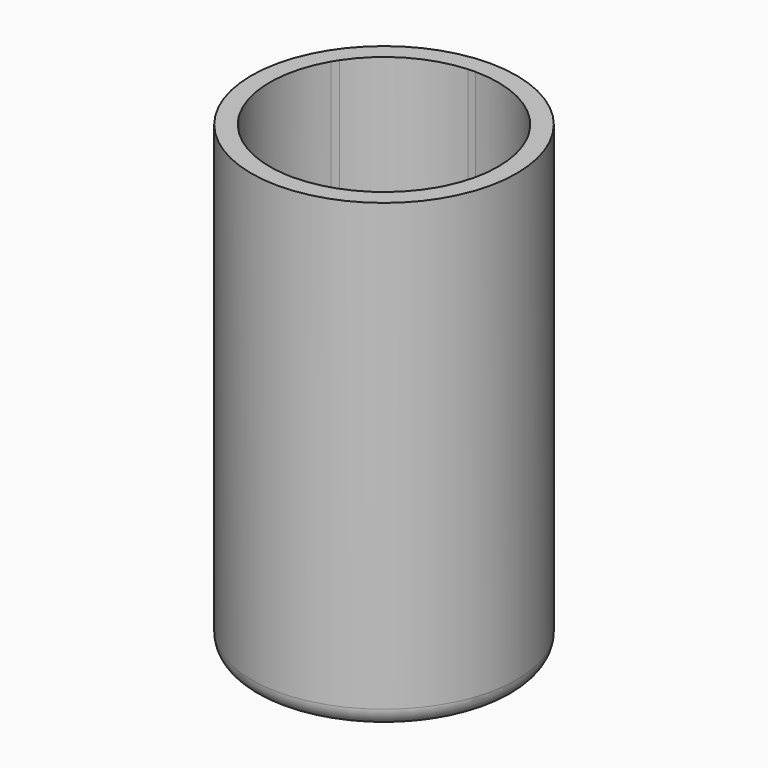
from build123d import *

# Parameters (mm, degrees)
F0_R     = 36
F1_DEPTH = 126
F2_DEPTH = 4
F3_R     = 5
F4_DEPTH = 10
F5_DEPTH = 5
F6_DEPTH = 5


# Not quite as in the source:
# - a feature names something its author has since deleted; it is built from what else it names


with BuildPart() as f1:
    # F0 (on Top) → F1 (new body)
    with BuildSketch(Plane.XY):
        Circle(F0_R)
        with BuildLine():
            ThreePointArc((27.7903944838, 13.7365925335), (30.1869361562, 7.0532889846), (31, 0))
            ThreePointArc((31, 0), (30.1869361562, -7.0532889846), (27.7903944838, -13.7365925335))
            ThreePointArc((27.7903944838, -13.7365925335), (27.33281573, -14.625907981), (26.8467875173, -15.5))
            ThreePointArc((26.8467875173, -15.5), (15.5, -26.8467875173), (0, -31))
            ThreePointArc((0, -31), (-1, -30.9838667697), (-1.9989591464, -30.935483871))
            ThreePointArc((-1.9989591464, -30.935483871), (-15.5, -26.8467875173), (-25.7914353374, -17.1988913374))
            ThreePointArc((-25.7914353374, -17.1988913374), (-26.33281573, -16.3579587886), (-26.8467875173, -15.5))
            ThreePointArc((-26.8467875173, -15.5), (-31, 0), (-26.8467875173, 15.5))
            ThreePointArc((-26.8467875173, 15.5), (-26.33281573, 16.3579587886), (-25.7914353374, 17.1988913374))
            ThreePointArc((-25.7914353374, 17.1988913374), (-15.5, 26.8467875173), (-1.9989591464, 30.935483871))
            ThreePointArc((-1.9989591464, 30.935483871), (-1, 30.9838667697), (0, 31))
            ThreePointArc((0, 31), (15.5, 26.8467875173), (26.8467875173, 15.5))
            ThreePointArc((26.8467875173, 15.5), (27.33281573, 14.625907981), (27.7903944838, 13.7365925335))
        make_face(mode=Mode.SUBTRACT)
    extrude(amount=F1_DEPTH)

    # F0 (on Top) → F2 (join)
    with BuildSketch(Plane.XY):
        with BuildLine():
            ThreePointArc((0, -31), (15.5, -26.8467875173), (26.8467875173, -15.5))
            Line((26.8467875173, -15.5), (22.5166604984, -13))
            ThreePointArc((22.5166604984, -13), (13, -22.5166604984), (0, -26))
            Line((0, -26), (0, -31))
        make_face()
        with BuildLine():
            ThreePointArc((0, -26), (13, -22.5166604984), (22.5166604984, -13))
            Line((22.5166604984, -13), (18.1865334795, -10.5))
            ThreePointArc((18.1865334795, -10.5), (10.5, -18.1865334795), (0, -21))
            Line((0, -21), (0, -26))
        make_face()
        with BuildLine():
            Line((-22.5166604984, 13), (-26.8467875173, 15.5))
            ThreePointArc((-26.8467875173, 15.5), (-31, 0), (-26.8467875173, -15.5))
            Line((-26.8467875173, -15.5), (-22.5166604984, -13))
            ThreePointArc((-22.5166604984, -13), (-26, 0), (-22.5166604984, 13))
        make_face()
        with BuildLine():
            Line((-18.1865334795, 10.5), (-22.5166604984, 13))
            ThreePointArc((-22.5166604984, 13), (-26, 0), (-22.5166604984, -13))
            Line((-22.5166604984, -13), (-18.1865334795, -10.5))
            ThreePointArc((-18.1865334795, -10.5), (-21, 0), (-18.1865334795, 10.5))
        make_face()
        with BuildLine():
            ThreePointArc((-26.8467875173, -15.5), (-26.33281573, -16.3579587886), (-25.7914353374, -17.1988913374))
            Line((-25.7914353374, -17.1988913374), (-21.631526412, -14.4248766056))
            ThreePointArc((-21.631526412, -14.4248766056), (-22.0855873864, -13.7195783388), (-22.5166604984, -13))
            Line((-22.5166604984, -13), (-26.8467875173, -15.5))
        make_face()
        with BuildLine():
            Line((0, 26), (0, 31))
            ThreePointArc((0, 31), (-1, 30.9838667697), (-1.9989591464, 30.935483871))
            Line((-1.9989591464, 30.935483871), (-1.6765463809, 25.9458896982))
            ThreePointArc((-1.6765463809, 25.9458896982), (-0.8387096774, 25.9864689036), (0, 26))
        make_face()
        with BuildLine():
            Line((22.5166604984, 13), (26.8467875173, 15.5))
            ThreePointArc((26.8467875173, 15.5), (15.5, 26.8467875173), (0, 31))
            Line((0, 31), (0, 26))
            ThreePointArc((0, 26), (13, 22.5166604984), (22.5166604984, 13))
        make_face()
        with BuildLine():
            Line((-1.6765463809, 25.9458896982), (-1.9989591464, 30.935483871))
            ThreePointArc((-1.9989591464, 30.935483871), (-15.5, 26.8467875173), (-25.7914353374, 17.1988913374))
            Line((-25.7914353374, 17.1988913374), (-21.631526412, 14.4248766056))
            ThreePointArc((-21.631526412, 14.4248766056), (-13, 22.5166604984), (-1.6765463809, 25.9458896982))
        make_face()
        with BuildLine():
            Line((18.1865334795, 10.5), (22.5166604984, 13))
            ThreePointArc((22.5166604984, 13), (13, 22.5166604984), (0, 26))
            Line((0, 26), (0, 21))
            ThreePointArc((0, 21), (10.5, 18.1865334795), (18.1865334795, 10.5))
        make_face()
        with BuildLine():
            Line((-21.631526412, 14.4248766056), (-25.7914353374, 17.1988913374))
            ThreePointArc((-25.7914353374, 17.1988913374), (-26.33281573, 16.3579587886), (-26.8467875173, 15.5))
            Line((-26.8467875173, 15.5), (-22.5166604984, 13))
            ThreePointArc((-22.5166604984, 13), (-22.0855873864, 13.7195783388), (-21.631526412, 14.4248766056))
        make_face()
        with BuildLine():
            Line((23.3080727929, 11.5210130927), (27.7903944838, 13.7365925335))
            ThreePointArc((27.7903944838, 13.7365925335), (27.33281573, 14.625907981), (26.8467875173, 15.5))
            Line((26.8467875173, 15.5), (22.5166604984, 13))
            ThreePointArc((22.5166604984, 13), (22.9242970639, 12.2668905647), (23.3080727929, 11.5210130927))
        make_face()
        with BuildLine():
            ThreePointArc((27.7903944838, -13.7365925335), (30.1869361562, -7.0532889846), (31, 0))
            ThreePointArc((31, 0), (30.1869361562, 7.0532889846), (27.7903944838, 13.7365925335))
            Line((27.7903944838, 13.7365925335), (23.3080727929, 11.5210130927))
            ThreePointArc((23.3080727929, 11.5210130927), (25.3180754859, 5.915661729), (26, 0))
            ThreePointArc((26, 0), (25.3180754859, -5.915661729), (23.3080727929, -11.5210130927))
            Line((23.3080727929, -11.5210130927), (27.7903944838, -13.7365925335))
        make_face()
        with BuildLine():
            ThreePointArc((26.8467875173, -15.5), (27.33281573, -14.625907981), (27.7903944838, -13.7365925335))
            Line((27.7903944838, -13.7365925335), (23.3080727929, -11.5210130927))
            ThreePointArc((23.3080727929, -11.5210130927), (22.9242970639, -12.2668905647), (22.5166604984, -13))
            Line((22.5166604984, -13), (26.8467875173, -15.5))
        make_face()
        with BuildLine():
            ThreePointArc((-1.9989591464, -30.935483871), (-1, -30.9838667697), (0, -31))
            Line((0, -31), (0, -26))
            ThreePointArc((0, -26), (-0.8387096774, -25.9864689036), (-1.6765463809, -25.9458896982))
            Line((-1.6765463809, -25.9458896982), (-1.9989591464, -30.935483871))
        make_face()
        with BuildLine():
            ThreePointArc((-25.7914353374, -17.1988913374), (-15.5, -26.8467875173), (-1.9989591464, -30.935483871))
            Line((-1.9989591464, -30.935483871), (-1.6765463809, -25.9458896982))
            ThreePointArc((-1.6765463809, -25.9458896982), (-13, -22.5166604984), (-21.631526412, -14.4248766056))
            Line((-21.631526412, -14.4248766056), (-25.7914353374, -17.1988913374))
        make_face()
    extrude(amount=F2_DEPTH)

    # F3
    f3_edges = [f1.edges().sort_by_distance(p)[0] for p in [
        (-36, 0, 0),
    ]]
    fillet(f3_edges, radius=F3_R)



with BuildPart() as f4:
    # F0 (on Top) → F4 (new body)
    with BuildSketch(Plane.XY):
        with BuildLine():
            ThreePointArc((26, 0), (25.3180754859, 5.915661729), (23.3080727929, 11.5210130927))
            Line((23.3080727929, 11.5210130927), (18.825751102, 9.3054336518))
            ThreePointArc((18.825751102, 9.3054336518), (20.4492148155, 4.7780344735), (21, 0))
            ThreePointArc((21, 0), (20.4492148155, -4.7780344735), (18.825751102, -9.3054336518))
            Line((18.825751102, -9.3054336518), (23.3080727929, -11.5210130927))
            ThreePointArc((23.3080727929, -11.5210130927), (25.3180754859, -5.915661729), (26, 0))
        make_face()
        with BuildLine():
            ThreePointArc((-21.631526412, -14.4248766056), (-13, -22.5166604984), (-1.6765463809, -25.9458896982))
            Line((-1.6765463809, -25.9458896982), (-1.3541336153, -20.9562955255))
            ThreePointArc((-1.3541336153, -20.9562955255), (-10.5, -18.1865334795), (-17.4716174866, -11.6508618737))
            Line((-17.4716174866, -11.6508618737), (-21.631526412, -14.4248766056))
        make_face()
        with BuildLine():
            Line((-1.3541336153, 20.9562955255), (-1.6765463809, 25.9458896982))
            ThreePointArc((-1.6765463809, 25.9458896982), (-13, 22.5166604984), (-21.631526412, 14.4248766056))
            Line((-21.631526412, 14.4248766056), (-17.4716174866, 11.6508618737))
            ThreePointArc((-17.4716174866, 11.6508618737), (-10.5, 18.1865334795), (-1.3541336153, 20.9562955255))
        make_face()
        with BuildLine():
            ThreePointArc((-15.8076539165, 10.541255981), (-9.5, 16.4544826719), (-1.2251685091, 18.9604578564))
            Line((-1.2251685091, 18.9604578564), (-1.3541336153, 20.9562955255))
            ThreePointArc((-1.3541336153, 20.9562955255), (-10.5, 18.1865334795), (-17.4716174866, 11.6508618737))
            Line((-17.4716174866, 11.6508618737), (-15.8076539165, 10.541255981))
        make_face()
        with BuildLine():
            Line((-1.3541336153, -20.9562955255), (-1.2251685091, -18.9604578564))
            ThreePointArc((-1.2251685091, -18.9604578564), (-9.5, -16.4544826719), (-15.8076539165, -10.541255981))
            Line((-15.8076539165, -10.541255981), (-17.4716174866, -11.6508618737))
            ThreePointArc((-17.4716174866, -11.6508618737), (-10.5, -18.1865334795), (-1.3541336153, -20.9562955255))
        make_face()
        with BuildLine():
            ThreePointArc((21, 0), (20.4492148155, 4.7780344735), (18.825751102, 9.3054336518))
            Line((18.825751102, 9.3054336518), (17.0328224256, 8.4192018754))
            ThreePointArc((17.0328224256, 8.4192018754), (18.5016705474, 4.3229835712), (19, 0))
            ThreePointArc((19, 0), (18.5016705474, -4.3229835712), (17.0328224256, -8.4192018754))
            Line((17.0328224256, -8.4192018754), (18.825751102, -9.3054336518))
            ThreePointArc((18.825751102, -9.3054336518), (20.4492148155, -4.7780344735), (21, 0))
        make_face()
    extrude(amount=F4_DEPTH)

    # F0 (on Top) → F5 (cut)
    with BuildSketch(Plane.XY):
        with BuildLine():
            ThreePointArc((-21.631526412, -14.4248766056), (-13, -22.5166604984), (-1.6765463809, -25.9458896982))
            Line((-1.6765463809, -25.9458896982), (-1.3541336153, -20.9562955255))
            ThreePointArc((-1.3541336153, -20.9562955255), (-10.5, -18.1865334795), (-17.4716174866, -11.6508618737))
            Line((-17.4716174866, -11.6508618737), (-21.631526412, -14.4248766056))
        make_face()
        with BuildLine():
            ThreePointArc((26, 0), (25.3180754859, 5.915661729), (23.3080727929, 11.5210130927))
            Line((23.3080727929, 11.5210130927), (18.825751102, 9.3054336518))
            ThreePointArc((18.825751102, 9.3054336518), (20.4492148155, 4.7780344735), (21, 0))
            ThreePointArc((21, 0), (20.4492148155, -4.7780344735), (18.825751102, -9.3054336518))
            Line((18.825751102, -9.3054336518), (23.3080727929, -11.5210130927))
            ThreePointArc((23.3080727929, -11.5210130927), (25.3180754859, -5.915661729), (26, 0))
        make_face()
        with BuildLine():
            Line((-1.3541336153, 20.9562955255), (-1.6765463809, 25.9458896982))
            ThreePointArc((-1.6765463809, 25.9458896982), (-13, 22.5166604984), (-21.631526412, 14.4248766056))
            Line((-21.631526412, 14.4248766056), (-17.4716174866, 11.6508618737))
            ThreePointArc((-17.4716174866, 11.6508618737), (-10.5, 18.1865334795), (-1.3541336153, 20.9562955255))
        make_face()
    extrude(amount=F5_DEPTH, mode=Mode.SUBTRACT)


with BuildPart() as f1_1:
    add(f1.part)

    add(f4.part)  # F6 merges F4
    # F0 (on Top) → F6 (join)
    with BuildSketch(Plane.XY):
        with BuildLine():
            Line((-1.2251685091, -18.9604578564), (0, 0))
            Line((0, 0), (-15.8076539165, -10.541255981))
            ThreePointArc((-15.8076539165, -10.541255981), (-9.5, -16.4544826719), (-1.2251685091, -18.9604578564))
        make_face()
        with BuildLine():
            ThreePointArc((-1.2251685091, -18.9604578564), (9.5, -16.4544826719), (17.0328224256, -8.4192018754))
            Line((17.0328224256, -8.4192018754), (0, 0))
            Line((0, 0), (-1.2251685091, -18.9604578564))
        make_face()
        with BuildLine():
            ThreePointArc((19, 0), (18.5016705474, 4.3229835712), (17.0328224256, 8.4192018754))
            Line((17.0328224256, 8.4192018754), (0, 0))
            Line((0, 0), (17.0328224256, -8.4192018754))
            ThreePointArc((17.0328224256, -8.4192018754), (18.5016705474, -4.3229835712), (19, 0))
        make_face()
        with BuildLine():
            Line((0, 0), (17.0328224256, 8.4192018754))
            ThreePointArc((17.0328224256, 8.4192018754), (9.5, 16.4544826719), (-1.2251685091, 18.9604578564))
            Line((-1.2251685091, 18.9604578564), (0, 0))
        make_face()
        with BuildLine():
            Line((0, 0), (-1.2251685091, 18.9604578564))
            ThreePointArc((-1.2251685091, 18.9604578564), (-9.5, 16.4544826719), (-15.8076539165, 10.541255981))
            Line((-15.8076539165, 10.541255981), (0, 0))
        make_face()
        with BuildLine():
            Line((-15.8076539165, -10.541255981), (0, 0))
            Line((0, 0), (-15.8076539165, 10.541255981))
            ThreePointArc((-15.8076539165, 10.541255981), (-19, 0), (-15.8076539165, -10.541255981))
        make_face()
        with BuildLine():
            Line((-1.3541336153, -20.9562955255), (-1.2251685091, -18.9604578564))
            ThreePointArc((-1.2251685091, -18.9604578564), (-9.5, -16.4544826719), (-15.8076539165, -10.541255981))
            Line((-15.8076539165, -10.541255981), (-17.4716174866, -11.6508618737))
            ThreePointArc((-17.4716174866, -11.6508618737), (-10.5, -18.1865334795), (-1.3541336153, -20.9562955255))
        make_face()
        with BuildLine():
            ThreePointArc((18.1865334795, -10.5), (18.5157783977, -9.9078731485), (18.825751102, -9.3054336518))
            Line((18.825751102, -9.3054336518), (17.0328224256, -8.4192018754))
            ThreePointArc((17.0328224256, -8.4192018754), (9.5, -16.4544826719), (-1.2251685091, -18.9604578564))
            Line((-1.2251685091, -18.9604578564), (-1.3541336153, -20.9562955255))
            ThreePointArc((-1.3541336153, -20.9562955255), (-0.6774193548, -20.9890710375), (0, -21))
            ThreePointArc((0, -21), (10.5, -18.1865334795), (18.1865334795, -10.5))
        make_face()
        with BuildLine():
            ThreePointArc((21, 0), (20.4492148155, 4.7780344735), (18.825751102, 9.3054336518))
            Line((18.825751102, 9.3054336518), (17.0328224256, 8.4192018754))
            ThreePointArc((17.0328224256, 8.4192018754), (18.5016705474, 4.3229835712), (19, 0))
            ThreePointArc((19, 0), (18.5016705474, -4.3229835712), (17.0328224256, -8.4192018754))
            Line((17.0328224256, -8.4192018754), (18.825751102, -9.3054336518))
            ThreePointArc((18.825751102, -9.3054336518), (20.4492148155, -4.7780344735), (21, 0))
        make_face()
        with BuildLine():
            Line((17.0328224256, 8.4192018754), (18.825751102, 9.3054336518))
            ThreePointArc((18.825751102, 9.3054336518), (18.5157783977, 9.9078731485), (18.1865334795, 10.5))
            ThreePointArc((18.1865334795, 10.5), (10.5, 18.1865334795), (0, 21))
            ThreePointArc((0, 21), (-0.6774193548, 20.9890710375), (-1.3541336153, 20.9562955255))
            Line((-1.3541336153, 20.9562955255), (-1.2251685091, 18.9604578564))
            ThreePointArc((-1.2251685091, 18.9604578564), (9.5, 16.4544826719), (17.0328224256, 8.4192018754))
        make_face()
        with BuildLine():
            ThreePointArc((-15.8076539165, 10.541255981), (-9.5, 16.4544826719), (-1.2251685091, 18.9604578564))
            Line((-1.2251685091, 18.9604578564), (-1.3541336153, 20.9562955255))
            ThreePointArc((-1.3541336153, 20.9562955255), (-10.5, 18.1865334795), (-17.4716174866, 11.6508618737))
            Line((-17.4716174866, 11.6508618737), (-15.8076539165, 10.541255981))
        make_face()
        with BuildLine():
            ThreePointArc((-15.8076539165, -10.541255981), (-19, 0), (-15.8076539165, 10.541255981))
            Line((-15.8076539165, 10.541255981), (-17.4716174866, 11.6508618737))
            ThreePointArc((-17.4716174866, 11.6508618737), (-17.8383590429, 11.0811978891), (-18.1865334795, 10.5))
            ThreePointArc((-18.1865334795, 10.5), (-21, 0), (-18.1865334795, -10.5))
            ThreePointArc((-18.1865334795, -10.5), (-17.8383590429, -11.0811978891), (-17.4716174866, -11.6508618737))
            Line((-17.4716174866, -11.6508618737), (-15.8076539165, -10.541255981))
        make_face()
    extrude(amount=-F6_DEPTH)


solid = f1_1.part
